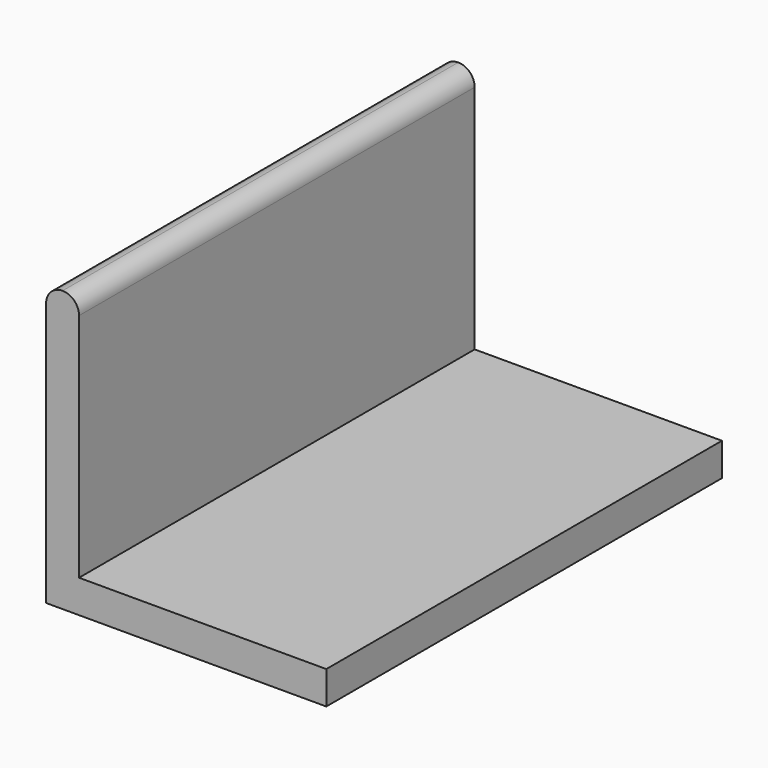
from build123d import *

# Parameters (mm, degrees)
F1_DEPTH = 60
F2_R     = 1.99999


# Not quite as in the source:
# - a fillet or chamfer is up to 0.001 mm smaller than in the source, because OpenCascade refuses the exact size


with BuildPart() as f1:
    # F0 (on Front) → F1 (new body)
    with BuildSketch(Plane.XZ):
        Polygon((0, 34), (0, 0), (34, 0), (34, 4), (4, 4), (4, 34), align=None)
    extrude(amount=F1_DEPTH)

    # F2 (radius 2 in the source; OpenCascade refuses exactly that, so slightly less here)
    f2_edges = [f1.edges().sort_by_distance(p)[0] for p in [
        (0, -30, 34),
        (4, -30, 34),
    ]]
    fillet(f2_edges, radius=F2_R)


solid = f1.part
